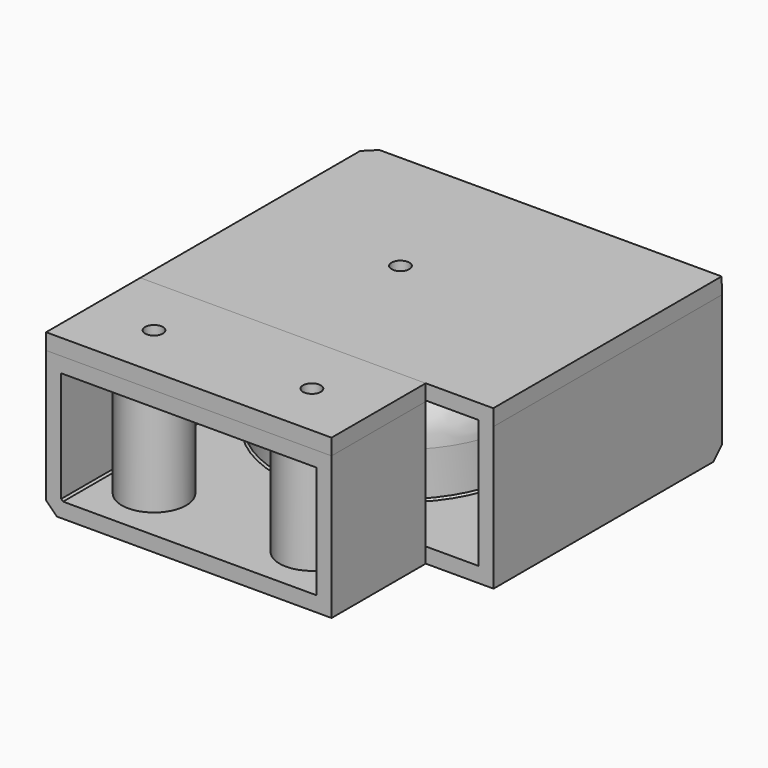
from build123d import *

# Parameters (mm, degrees)
F0_W      = 80
F0_H      = 40
F1_DEPTH  = 113
F0_H_2    = 4.5
F2_DEPTH  = 80
F3_R      = 30
F4_DEPTH  = 32
F5_R      = 2.499995835
F5_R_2    = 2.5
F6_DEPTH  = 44.501
F7_R      = 15
F8_SIZE   = 3
F5_R_3    = 4.8
F5_R_4    = 4.799995835
F9_DEPTH  = 31.5
F10_T     = 4.25
F11_DEPTH = 4.5
F12_DEPTH = 35


# Not quite as in the source:
# - a shell that OpenCascade refuses in one call is made with other operations: the cavity is built on its own and cut out


with BuildPart() as f1:
    # F0 (on Front) → F1 (new body)
    with BuildSketch(Plane.XZ):
        with Locations((-0.921532978, 11.1246381328)):
            Rectangle(F0_W, F0_H)
    extrude(amount=F1_DEPTH)

    # F0 (on Front) → F2 (join)
    with BuildSketch(Plane.XZ):
        with Locations((-0.921532978, 33.3746381328)):
            Rectangle(F0_W, F0_H_2)
        Polygon((39.078467022, 31.1246381328), (39.078467022, -8.8753618672), (58.078467022, -8.8753618672), (58.078467022, 31.1246381328), (57.9992160201, 35.6246381328), (39.078467022, 35.6246381328), align=None)
    extrude(amount=F2_DEPTH)

    # F3 (on face) → F4 (cut)
    with BuildSketch(Plane(origin=(0, 0, -8.8753618672), x_dir=(1, 0, 0), z_dir=(0, 0, -1))):
        with Locations((0, 40)):
            Circle(F3_R)
    extrude(amount=-F4_DEPTH, mode=Mode.SUBTRACT)

    # F5 (on face) → F6 (cut, through all)
    with BuildSketch(Plane(origin=(0, 0, -8.8753618672), x_dir=(1, 0, 0), z_dir=(0, 0, -1))):
        with Locations((-23.0447813567, 97.5387539414)):
            Circle(F5_R)
        with Locations((21.201467022, 97.5387539414)):
            Circle(F5_R_2)
        with Locations((0, 40)):
            Circle(F5_R_2)
    extrude(amount=-F6_DEPTH, mode=Mode.SUBTRACT)

    # F7
    f7_edges = [f1.edges().sort_by_distance(p)[0] for p in [
        (-30, -40, 23.124638),
    ]]
    fillet(f7_edges, radius=F7_R)

    # F8
    f8_edges = [f1.edges().sort_by_distance(p)[0] for p in [
        (-30, -40, -8.875362),
        (-40.921533, -56.5, -8.875362),
        (-40.921533, 0, 13.374638),
        (8.578467, 0, -8.875362),
        (18.701467, -97.538754, -8.875362),
        (-25.544777, -97.538754, -8.875362),
    ]]
    chamfer(f8_edges, length=F8_SIZE)

    # F5 (on face) → F9 (cut)
    with BuildSketch(Plane(origin=(0, 0, -8.8753618672), x_dir=(1, 0, 0), z_dir=(0, 0, -1))):
        with Locations((21.201467022, 97.5387539414)):
            Circle(F5_R_3)
        with Locations((21.201467022, 97.5387539414)):
            Circle(F5_R_2, mode=Mode.SUBTRACT)
        with Locations((-23.0447813567, 97.5387539414)):
            Circle(F5_R_4)
        with Locations((-23.0447813567, 97.5387539414)):
            Circle(F5_R, mode=Mode.SUBTRACT)
    extrude(amount=-F9_DEPTH, mode=Mode.SUBTRACT)

    # F10: shell of thickness 4.25, made by hand


with BuildPart() as f10_core1:
    # F10_t2: copy of F1
    add(f1.part)

    # the walls: a layer under each face that stays
    f10_faces = [f10_core1.faces().sort_by_distance(p)[0] for p in [
        (-30, -40, 1.1246381328),
        (-31.5, -40, -7.3753618672),
        (-25.6066017178, -40, 18.7312398505),
        (10.078467022, -94.6666666667, -8.8753618672),
        (-10, -30, 23.1246381328),
        (58.078467022, -40, 11.1246381328),
        (10.078467022, -1.5, -7.3753618672),
        (-39.421532978, -58, -7.3753618672),
        (39.078467022, -96.5, 11.1246381328),
        (16.051467022, -97.5387539414, -8.5253618672),
        (-28.1947771917, -97.5387539414, -8.5253618672),
        (-2.5, -40, 29.3746381328),
        (10.078467022, 0, 14.8746381328),
        (58.0388415211, -40, 33.3746381328),
        (-38.671532978, -1.5, -6.6253618672),
        (-40.921532978, -58, 14.8746381328),
        (-0.921532978, -96.5, 31.1246381328),
        (8.5388415211, -40, 35.6246381328),
        (16.401467022, -97.5387539414, 7.2246381328),
        (-27.8447771917, -97.5387539414, 7.2246381328),
        (-39.421532978, -1.5, 14.8746381328),
        (18.701467022, -97.5387539414, 26.8746381328),
        (-25.5447771917, -97.5387539414, 26.8746381328),
        (18.001467022, -94.3387539414, 22.6246381328),
        (-26.2447785801, -94.338756718, 22.6246381328),
    ]]
    thicken(f10_faces, amount=-F10_T, mode=Mode.SUBTRACT)

    # F10_s3 → F10_t4 (revolve, cut)
    with BuildSketch(Plane.XZ.offset(97.5387539414)):
        Polygon((25.958967022, 22.5821381328), (30.251467022, 22.6246381328), (30.251467022, 26.8746381328), (26.001467022, 26.8746381328), align=None)
    revolve(axis=Axis((21.201467022, -97.5387539414, 22.6246381328), (0, 0, -1)), mode=Mode.SUBTRACT)

    # F10_s5 → F10_t6 (revolve, cut)
    with BuildSketch(Plane.XZ.offset(97.5387539414)):
        Polygon((-18.2872855217, 22.5821381328), (-13.9947855217, 22.6246381328), (-13.9947855217, 26.8746381328), (-18.2447855217, 26.8746381328), align=None)
    revolve(axis=Axis((-23.0447813567, -97.5387539414, 22.6246381328), (0, 0, -1)), mode=Mode.SUBTRACT)


with BuildPart() as f1_1:
    add(f1.part)

    # what is left inside the walls is the cavity
    f10_cavity = [f10_core1.part.solids().sort_by_distance(p)[0] for p in [
        (8.575936, -54.75, 31.332138),
    ]]
    add(f10_cavity, mode=Mode.SUBTRACT)


with BuildPart() as f11:
    # F11 (new): a face of the model
    f11_faces = [f1_1.part.faces().sort_by_distance(p)[0] for p in [
        (-0.9215316593, -96.4843152878, 31.1246381328),
    ]]
    extrude(f11_faces, amount=F11_DEPTH)


with BuildPart() as f1_2:
    add(f1_1.part)

    # F5 (on face) → F12 (cut)
    with BuildSketch(Plane(origin=(0, 0, -8.8753618672), x_dir=(1, 0, 0), z_dir=(0, 0, -1))):
        with Locations((0, 40)):
            Circle(F5_R_3)
        with Locations((0, 40)):
            Circle(F5_R_2, mode=Mode.SUBTRACT)
    extrude(amount=-F12_DEPTH, mode=Mode.SUBTRACT)


solid = Compound([f11.part, f1_2.part])
